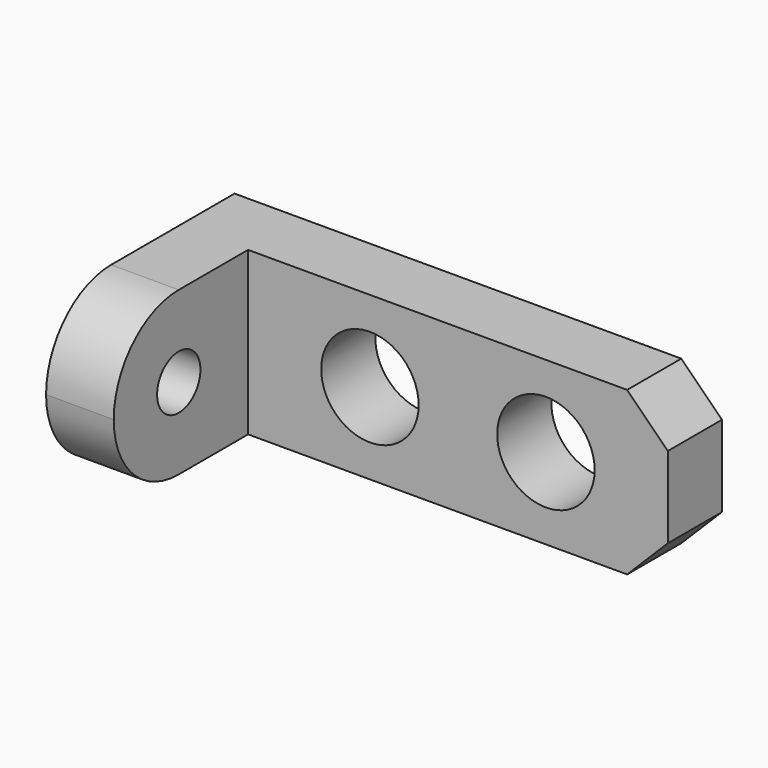
from build123d import *

# Parameters (mm, degrees)
F0_W     = 4572
F0_H     = 1524
F1_DEPTH = 635
F2_W     = 635
F2_H     = 1524
F3_DEPTH = 1574.8
F4_R     = 761.99999
F5_R     = 457.2
F6_DEPTH = 635
F7_R     = 254
F8_DEPTH = 635.001
F9_SIZE  = 381


# Not quite as in the source:
# - a fillet or chamfer is up to 0.001 mm smaller than in the source, because OpenCascade refuses the exact size


with BuildPart() as f1:
    # F0 (on Front) → F1 (new body)
    with BuildSketch(Plane.XZ):
        Rectangle(F0_W, F0_H)
    extrude(amount=F1_DEPTH)

    # F2 (on face) → F3 (join)
    with BuildSketch(Plane.XZ.offset(635)):
        with Locations((-1968.5, 0)):
            Rectangle(F2_W, F2_H)
    extrude(amount=F3_DEPTH)

    # F4 (radius 762 in the source; OpenCascade refuses exactly that, so slightly less here)
    f4_edges = [f1.edges().sort_by_distance(p)[0] for p in [
        (-1968.5, -2209.8, 762),
        (-1968.5, -2209.8, -762),
    ]]
    fillet(f4_edges, radius=F4_R)

    # F5 (on face) → F6 (cut)
    with BuildSketch(Plane.XZ.offset(635)):
        with Locations((-508, 0)):
            Circle(F5_R)
        with Locations((1143, 0)):
            Circle(F5_R)
    extrude(amount=-F6_DEPTH, mode=Mode.SUBTRACT)

    # F7 (on face) → F8 (cut, through all)
    with BuildSketch(Plane.YZ.offset(-1651)):
        with Locations((-1447.8, 0)):
            Circle(F7_R)
    extrude(amount=-F8_DEPTH, mode=Mode.SUBTRACT)

    # F9
    f9_edges = [f1.edges().sort_by_distance(p)[0] for p in [
        (2286, -317.5, -762),
        (2286, -317.5, 762),
    ]]
    chamfer(f9_edges, length=F9_SIZE)


solid = f1.part
